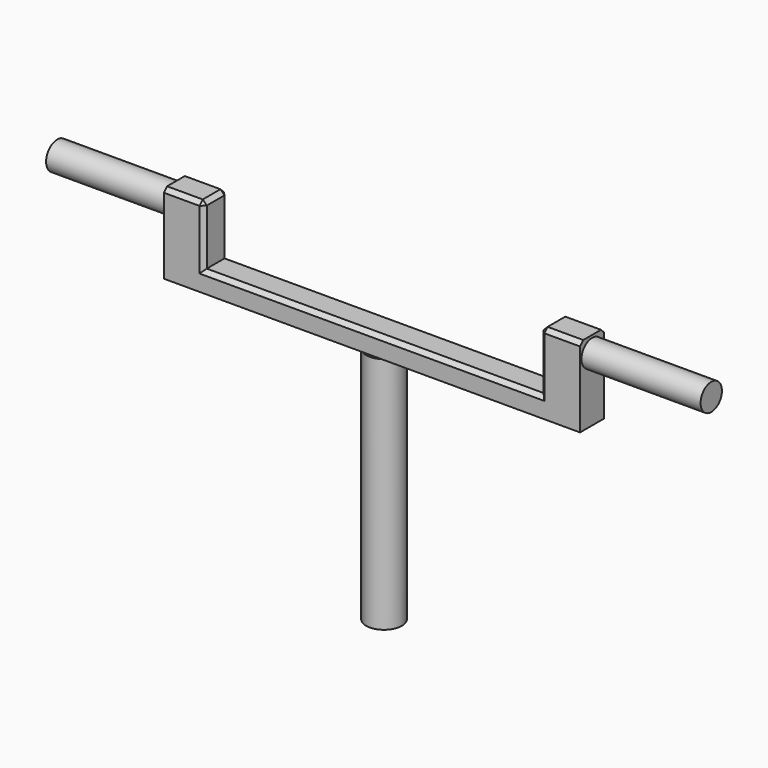
from build123d import *

# Parameters (mm, degrees)
F0_R      = 22.5
F1_DEPTH  = 300
F2_W      = 24.0328347509
F2_H      = 38.0450108928
F3_DEPTH  = 25.4
F4_W      = 38.0450108928
F4_H      = 25.4
F5_DEPTH  = 250
F6_W      = 50
F6_H      = 38.0450108928
F7_DEPTH  = 75
F9_W      = 38.0450108928
F9_H      = 25.4
F10_DEPTH = 250
F11_W     = 50
F11_H     = 38.0450108928
F12_DEPTH = 75
F13_R     = 16.7747006108
F14_DEPTH = 150
F8_R      = 17.5763954382
F15_DEPTH = 150
F16_SIZE  = 5.08


with BuildPart() as f1:
    # F0 (on Top) → F1 (new body)
    with BuildSketch(Plane.XY):
        with Locations((-6.6593382508, 15.5711015686)):
            Circle(F0_R)
    extrude(amount=F1_DEPTH)

    # F2 (on face) → F3 (join)
    with BuildSketch(Plane.XY.offset(300)):
        with Locations((-6.6593382508, 15.5711015686)):
            Rectangle(F2_W, F2_H)
    extrude(amount=F3_DEPTH)

    # F4 (on face) → F5 (join)
    with BuildSketch(Plane(origin=(-18.6757556262, 0, 0), x_dir=(0, -1, 0), z_dir=(-1, 0, 0))):
        with Locations((-15.5711015686, 312.7)):
            Rectangle(F4_W, F4_H)
    extrude(amount=F5_DEPTH)

    # F6 (on face) → F7 (join)
    with BuildSketch(Plane.XY.offset(325.4)):
        with Locations((-243.6757556262, 15.5711015686)):
            Rectangle(F6_W, F6_H)
    extrude(amount=F7_DEPTH)

    # F9 (on face) → F10 (join)
    with BuildSketch(Plane.YZ.offset(5.3570791247)):
        with Locations((15.5711015686, 312.7)):
            Rectangle(F9_W, F9_H)
    extrude(amount=F10_DEPTH)

    # F11 (on face) → F12 (join)
    with BuildSketch(Plane.XY.offset(325.4)):
        with Locations((230.3570791247, 15.5711015686)):
            Rectangle(F11_W, F11_H)
    extrude(amount=F12_DEPTH)

    # F13 (on face) → F14 (join)
    with BuildSketch(Plane.YZ.offset(255.3570791247)):
        with Locations((15.5711015686, 380.4)):
            Circle(F13_R)
    extrude(amount=F14_DEPTH)

    # F8 (on face) → F15 (join)
    with BuildSketch(Plane(origin=(-268.6757556262, 0, 0), x_dir=(0, -1, 0), z_dir=(-1, 0, 0))):
        with Locations((-16.2542480975, 380.010843277)):
            Circle(F8_R)
    extrude(amount=F15_DEPTH)

    # F16
    f16_edges = [f1.edges().sort_by_distance(p)[0] for p in [
        (-6.659338, -3.451404, 325.4),
        (-6.659338, 34.593607, 325.4),
        (-218.675756, -3.451404, 362.9),
        (-218.675756, 34.593607, 362.9),
        (205.357079, -3.451404, 362.9),
        (205.357079, 34.593607, 362.9),
        (205.357079, 15.571102, 400.4),
        (-218.675756, 15.571102, 400.4),
        (-243.675756, -3.451404, 400.4),
        (-243.675756, 34.593607, 400.4),
        (230.357079, 34.593607, 400.4),
        (230.357079, -3.451404, 400.4),
    ]]
    chamfer(f16_edges, length=F16_SIZE)


solid = f1.part
